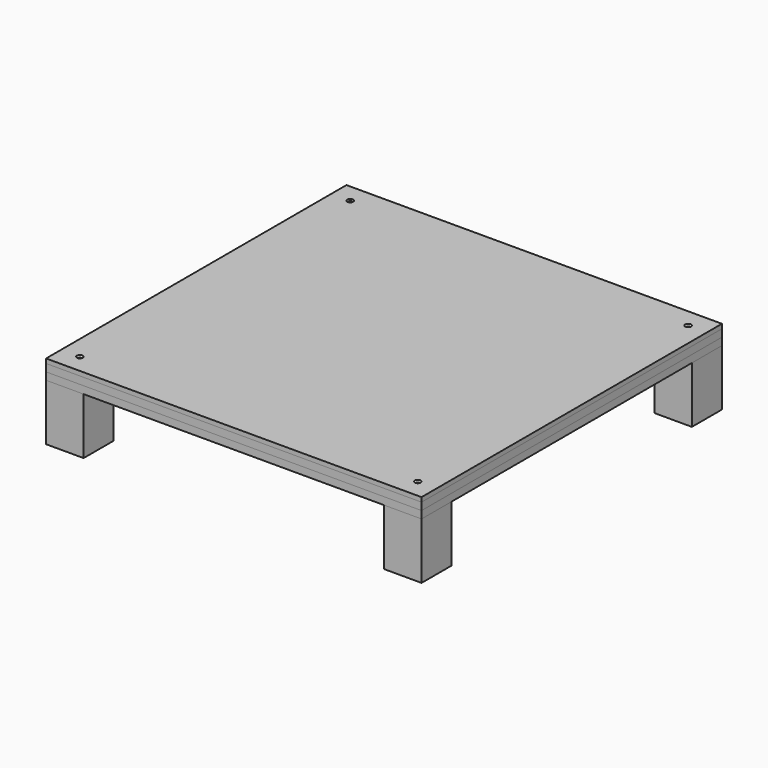
from build123d import *

# Parameters (mm, degrees)
F1_W            = 254
F1_H            = 254
F2_DEPTH        = 4.99999
F0_W            = 254
F0_H            = 254
F3_DEPTH        = 2.999994
F4_DEPTH        = 4.99999
F5_W            = 25.4
F5_H            = 25.4
F6_DEPTH        = 38.1
F7_W            = 25.4
F7_H            = 25.4
F8_DEPTH        = 38.1
F9_W            = 25.4
F9_H            = 25.4
F10_DEPTH       = 38.1
F11_W           = 25.4
F11_H           = 25.4
F12_DEPTH       = 38.1
F14_D           = 2.4892
F14_DEPTH       = 25.4
F14_TIP         = 0.7478311264
F14_2_D         = 2.4892
F14_2_DEPTH     = 25.4
F14_2_TIP       = 0.7478311264
F14_3_D         = 2.4892
F14_3_DEPTH     = 25.4
F14_3_TIP       = 0.7478311264
F14_4_D         = 2.4892
F14_4_DEPTH     = 25.4
F14_4_TIP       = 0.7478311264
F16_D           = 2.4892
F16_DEPTH       = 3.999992
F16_CSINK_D     = 3.999992
F16_CSINK_ANGLE = 90
F16_TIP         = 0.7478311264
F18_D           = 2.00000108
F18_DEPTH       = 25.4
F18_TIP         = 0.6008609435
F18_2_D         = 2.00000108
F18_2_DEPTH     = 25.4
F18_2_TIP       = 0.6008609435
F18_3_D         = 2.00000108
F18_3_DEPTH     = 25.4
F18_3_TIP       = 0.6008609435
F18_4_D         = 2.00000108
F18_4_DEPTH     = 25.4
F18_4_TIP       = 0.6008609435
F20_D           = 2.00000108
F20_DEPTH       = 3.999992
F20_CSINK_D     = 3.999992
F20_CSINK_ANGLE = 90
F20_TIP         = 0.6008609435
F22_D           = 2
F22_DEPTH       = 25.4
F22_TIP         = 0.600860619
F22_2_D         = 2
F22_2_DEPTH     = 25.4
F22_2_TIP       = 0.600860619
F22_3_D         = 2
F22_3_DEPTH     = 25.4
F22_3_TIP       = 0.600860619
F22_4_D         = 2
F22_4_DEPTH     = 25.4
F22_4_TIP       = 0.600860619
F23_D           = 2
F23_DEPTH       = 25.4
F23_TIP         = 0.600860619
F23_2_D         = 2
F23_2_DEPTH     = 25.4
F23_2_TIP       = 0.600860619
F23_3_D         = 2
F23_3_DEPTH     = 25.4
F23_3_TIP       = 0.600860619
F23_4_D         = 2
F23_4_DEPTH     = 25.4
F23_4_TIP       = 0.600860619
F24_D           = 2
F24_DEPTH       = 4
F24_CSINK_D     = 4
F24_CSINK_ANGLE = 90
F24_TIP         = 0.600860619
F25_D           = 2
F25_DEPTH       = 4
F25_CSINK_D     = 4
F25_CSINK_ANGLE = 90
F25_TIP         = 0.600860619
F26_W           = 203.2
F26_H           = 203.2
F27_DEPTH       = 5
F28_W           = 25.4
F28_H           = 25.4
F29_DEPTH       = 5
F30_W           = 25.4
F30_H           = 25.4
F31_DEPTH       = 5
F32_W           = 25.4
F32_H           = 25.4
F33_DEPTH       = 5
F34_W           = 25.4
F34_H           = 25.4
F35_DEPTH       = 5
F36_W           = 25.4
F36_H           = 25.4
F37_DEPTH       = 5


with BuildPart() as f2:
    # F1 (on Top) → F2 (new body)
    with BuildSketch(Plane.XY):
        Rectangle(F1_W, F1_H)
    extrude(amount=-F2_DEPTH)


with BuildPart() as f3:
    # F0 (on Top) → F3 (new body)
    with BuildSketch(Plane.XY):
        Rectangle(F0_W, F0_H)
    extrude(amount=F3_DEPTH)

    # F14#2
    with Locations(Plane.XY.offset(2.999994)):
        with Locations((-114.3, 114.3)):
            Hole(F14_2_D / 2, depth=F14_2_DEPTH)
            with Locations((0, 0, -(F14_2_DEPTH + F14_2_TIP / 2))):  # 118° drill point
                Cone(0, F14_2_D / 2, F14_2_TIP, mode=Mode.SUBTRACT)

    # F16
    with Locations(Plane.XY.offset(2.999994)):
        with Locations((-114.3, 114.3)):
            CounterSinkHole(F16_D / 2, F16_CSINK_D / 2, depth=F16_DEPTH, counter_sink_angle=F16_CSINK_ANGLE)
            with Locations((0, 0, -(F16_DEPTH + F16_TIP / 2))):  # 118° drill point
                Cone(0, F16_D / 2, F16_TIP, mode=Mode.SUBTRACT)

    # F18#2
    with Locations(Plane.XY.offset(2.999994)):
        with Locations((114.3, 114.3)):
            Hole(F18_2_D / 2, depth=F18_2_DEPTH)
            with Locations((0, 0, -(F18_2_DEPTH + F18_2_TIP / 2))):  # 118° drill point
                Cone(0, F18_2_D / 2, F18_2_TIP, mode=Mode.SUBTRACT)

    # F20
    with Locations(Plane.XY.offset(2.999994)):
        with Locations((114.3, 114.3)):
            CounterSinkHole(F20_D / 2, F20_CSINK_D / 2, depth=F20_DEPTH, counter_sink_angle=F20_CSINK_ANGLE)
            with Locations((0, 0, -(F20_DEPTH + F20_TIP / 2))):  # 118° drill point
                Cone(0, F20_D / 2, F20_TIP, mode=Mode.SUBTRACT)

    # F22#2
    with Locations(Plane.XY.offset(2.999994)):
        with Locations((-114.3, -114.3)):
            Hole(F22_2_D / 2, depth=F22_2_DEPTH)
            with Locations((0, 0, -(F22_2_DEPTH + F22_2_TIP / 2))):  # 118° drill point
                Cone(0, F22_2_D / 2, F22_2_TIP, mode=Mode.SUBTRACT)

    # F23#2
    with Locations(Plane.XY.offset(2.999994)):
        with Locations((114.3, -114.3)):
            Hole(F23_2_D / 2, depth=F23_2_DEPTH)
            with Locations((0, 0, -(F23_2_DEPTH + F23_2_TIP / 2))):  # 118° drill point
                Cone(0, F23_2_D / 2, F23_2_TIP, mode=Mode.SUBTRACT)

    # F24
    with Locations(Plane.XY.offset(2.999994)):
        with Locations((114.3, -114.3)):
            CounterSinkHole(F24_D / 2, F24_CSINK_D / 2, depth=F24_DEPTH, counter_sink_angle=F24_CSINK_ANGLE)
            with Locations((0, 0, -(F24_DEPTH + F24_TIP / 2))):  # 118° drill point
                Cone(0, F24_D / 2, F24_TIP, mode=Mode.SUBTRACT)

    # F25
    with Locations(Plane.XY.offset(2.999994)):
        with Locations((-114.3, -114.3)):
            CounterSinkHole(F25_D / 2, F25_CSINK_D / 2, depth=F25_DEPTH, counter_sink_angle=F25_CSINK_ANGLE)
            with Locations((0, 0, -(F25_DEPTH + F25_TIP / 2))):  # 118° drill point
                Cone(0, F25_D / 2, F25_TIP, mode=Mode.SUBTRACT)


with BuildPart() as f4:
    # F4 (new): a face of the model
    f4_faces = [f2.part.faces().sort_by_distance(p)[0] for p in [
        (0, 0, -4.99999),
    ]]
    extrude(f4_faces, amount=F4_DEPTH)

    # F14#3
    with Locations(Plane.XY.offset(2.999994)):
        with Locations((-114.3, 114.3)):
            Hole(F14_3_D / 2, depth=F14_3_DEPTH)
            with Locations((0, 0, -(F14_3_DEPTH + F14_3_TIP / 2))):  # 118° drill point
                Cone(0, F14_3_D / 2, F14_3_TIP, mode=Mode.SUBTRACT)

    # F18#3
    with Locations(Plane.XY.offset(2.999994)):
        with Locations((114.3, 114.3)):
            Hole(F18_3_D / 2, depth=F18_3_DEPTH)
            with Locations((0, 0, -(F18_3_DEPTH + F18_3_TIP / 2))):  # 118° drill point
                Cone(0, F18_3_D / 2, F18_3_TIP, mode=Mode.SUBTRACT)

    # F22#3
    with Locations(Plane.XY.offset(2.999994)):
        with Locations((-114.3, -114.3)):
            Hole(F22_3_D / 2, depth=F22_3_DEPTH)
            with Locations((0, 0, -(F22_3_DEPTH + F22_3_TIP / 2))):  # 118° drill point
                Cone(0, F22_3_D / 2, F22_3_TIP, mode=Mode.SUBTRACT)

    # F23#3
    with Locations(Plane.XY.offset(2.999994)):
        with Locations((114.3, -114.3)):
            Hole(F23_3_D / 2, depth=F23_3_DEPTH)
            with Locations((0, 0, -(F23_3_DEPTH + F23_3_TIP / 2))):  # 118° drill point
                Cone(0, F23_3_D / 2, F23_3_TIP, mode=Mode.SUBTRACT)


with BuildPart() as f6:
    # F5 (on face) → F6 (new body)
    with BuildSketch(Plane(origin=(0, 0, -9.99998), x_dir=(1, 0, 0), z_dir=(0, 0, -1))):
        with Locations((-114.3, 114.3)):
            Rectangle(F5_W, F5_H)
    extrude(amount=F6_DEPTH)

    # F22#4
    with Locations(Plane.XY.offset(2.999994)):
        with Locations((-114.3, -114.3)):
            Hole(F22_4_D / 2, depth=F22_4_DEPTH)
            with Locations((0, 0, -(F22_4_DEPTH + F22_4_TIP / 2))):  # 118° drill point
                Cone(0, F22_4_D / 2, F22_4_TIP, mode=Mode.SUBTRACT)


with BuildPart() as f8:
    # F7 (on face) → F8 (new body)
    with BuildSketch(Plane(origin=(0, 0, -9.99998), x_dir=(1, 0, 0), z_dir=(0, 0, -1))):
        with Locations((114.3, 114.3)):
            Rectangle(F7_W, F7_H)
    extrude(amount=F8_DEPTH)

    # F23#4
    with Locations(Plane.XY.offset(2.999994)):
        with Locations((114.3, -114.3)):
            Hole(F23_4_D / 2, depth=F23_4_DEPTH)
            with Locations((0, 0, -(F23_4_DEPTH + F23_4_TIP / 2))):  # 118° drill point
                Cone(0, F23_4_D / 2, F23_4_TIP, mode=Mode.SUBTRACT)


with BuildPart() as f10:
    # F9 (on face) → F10 (new body)
    with BuildSketch(Plane(origin=(0, 0, -9.99998), x_dir=(1, 0, 0), z_dir=(0, 0, -1))):
        with Locations((114.3, -114.3)):
            Rectangle(F9_W, F9_H)
    extrude(amount=F10_DEPTH)

    # F18#4
    with Locations(Plane.XY.offset(2.999994)):
        with Locations((114.3, 114.3)):
            Hole(F18_4_D / 2, depth=F18_4_DEPTH)
            with Locations((0, 0, -(F18_4_DEPTH + F18_4_TIP / 2))):  # 118° drill point
                Cone(0, F18_4_D / 2, F18_4_TIP, mode=Mode.SUBTRACT)


with BuildPart() as f12:
    # F11 (on face) → F12 (new body)
    with BuildSketch(Plane(origin=(0, 0, -9.99998), x_dir=(1, 0, 0), z_dir=(0, 0, -1))):
        with Locations((-114.3, -114.3)):
            Rectangle(F11_W, F11_H)
    extrude(amount=F12_DEPTH)

    # F14#4
    with Locations(Plane.XY.offset(2.999994)):
        with Locations((-114.3, 114.3)):
            Hole(F14_4_D / 2, depth=F14_4_DEPTH)
            with Locations((0, 0, -(F14_4_DEPTH + F14_4_TIP / 2))):  # 118° drill point
                Cone(0, F14_4_D / 2, F14_4_TIP, mode=Mode.SUBTRACT)


with BuildPart() as f2_1:
    add(f2.part)

    # F14
    with Locations(Plane.XY.offset(2.999994)):
        with Locations((-114.3, 114.3)):
            Hole(F14_D / 2, depth=F14_DEPTH)
            with Locations((0, 0, -(F14_DEPTH + F14_TIP / 2))):  # 118° drill point
                Cone(0, F14_D / 2, F14_TIP, mode=Mode.SUBTRACT)

    # F18
    with Locations(Plane.XY.offset(2.999994)):
        with Locations((114.3, 114.3)):
            Hole(F18_D / 2, depth=F18_DEPTH)
            with Locations((0, 0, -(F18_DEPTH + F18_TIP / 2))):  # 118° drill point
                Cone(0, F18_D / 2, F18_TIP, mode=Mode.SUBTRACT)

    # F22
    with Locations(Plane.XY.offset(2.999994)):
        with Locations((-114.3, -114.3)):
            Hole(F22_D / 2, depth=F22_DEPTH)
            with Locations((0, 0, -(F22_DEPTH + F22_TIP / 2))):  # 118° drill point
                Cone(0, F22_D / 2, F22_TIP, mode=Mode.SUBTRACT)

    # F23
    with Locations(Plane.XY.offset(2.999994)):
        with Locations((114.3, -114.3)):
            Hole(F23_D / 2, depth=F23_DEPTH)
            with Locations((0, 0, -(F23_DEPTH + F23_TIP / 2))):  # 118° drill point
                Cone(0, F23_D / 2, F23_TIP, mode=Mode.SUBTRACT)


with BuildPart() as f27_tool:
    # F26 (on face) → F27 (new body)
    with BuildSketch(Plane.XY):
        Rectangle(F26_W, F26_H)
    extrude(amount=-F27_DEPTH)


with BuildPart() as f2_2:
    add(f2_1.part)

    # F27: cut by f27_tool
    add(f27_tool.part, mode=Mode.SUBTRACT)


with BuildPart() as f4_1:
    add(f4.part)

    # F27: cut by f27_tool
    add(f27_tool.part, mode=Mode.SUBTRACT)


with BuildPart() as f29:
    # F28 (on face) → F29 (new body)
    with BuildSketch(Plane.XY):
        with Locations((-12.7, -12.7)):
            Rectangle(F28_W, F28_H)
    extrude(amount=-F29_DEPTH)


with BuildPart() as f31:
    # F30 (on face) → F31 (new body)
    with BuildSketch(Plane.XY):
        with Locations((-12.7, 12.7)):
            Rectangle(F30_W, F30_H)
    extrude(amount=-F31_DEPTH)


with BuildPart() as f33:
    # F32 (on face) → F33 (new body)
    with BuildSketch(Plane.XY):
        with Locations((12.7, -12.7)):
            Rectangle(F32_W, F32_H)
    extrude(amount=-F33_DEPTH)


with BuildPart() as f35:
    # F34 (on face) → F35 (new body)
    with BuildSketch(Plane.XY):
        with Locations((38.1, -38.1)):
            Rectangle(F34_W, F34_H)
    extrude(amount=-F35_DEPTH)


with BuildPart() as f37:
    # F36 (on face) → F37 (new body)
    with BuildSketch(Plane.XY):
        with Locations((12.7, 12.7)):
            Rectangle(F36_W, F36_H)
    extrude(amount=-F37_DEPTH)


with BuildPart() as f38_1:
    # F38: copy of F37
    add(f37.part.moved(Location((25.4, 25.4, 0))))


with BuildPart() as f39_1:
    # F39: copy of F38_1
    add(f38_1.part.moved(Location((25.4, 25.4, 0))))


with BuildPart() as f40_1:
    # F40: copy of F39_1
    add(f39_1.part.moved(Location((25.4, 25.4, 0))))


with BuildPart() as f41_1:
    # F41: copy of F29
    add(f29.part.moved(Location((-25.4, -25.4, 0))))


with BuildPart() as f42_1:
    # F42: copy of F41_1
    add(f41_1.part.moved(Location((-25.4, -25.4, 0))))


with BuildPart() as f43_1:
    # F43: copy of F42_1
    add(f42_1.part.moved(Location((-25.4, -25.4, 0))))


with BuildPart() as f44_1:
    # F44: copy of F31
    add(f31.part.moved(Location((-25.4, 25.4, 0))))


with BuildPart() as f45_1:
    # F45: copy of F44_1
    add(f44_1.part.moved(Location((-25.4, 25.4, 0))))


with BuildPart() as f46_1:
    # F46: copy of F45_1
    add(f45_1.part.moved(Location((-25.4, 25.4, 0))))


with BuildPart() as f47_1:
    # F47: copy of F35
    add(f35.part.moved(Location((25.4, -25.4, 0))))


with BuildPart() as f48_1:
    # F48: copy of F47_1
    add(f47_1.part.moved(Location((25.4, -25.4, 0))))


with BuildPart() as f49_1:
    # F49: copy of F48_1
    add(f48_1.part.moved(Location((-50.8, 0, 0))))


with BuildPart() as f50_1:
    # F50: copy of F49_1
    add(f49_1.part.moved(Location((-50.8, 0, 0))))


with BuildPart() as f51_1:
    # F51: copy of F50_1
    add(f50_1.part.moved(Location((-50.8, 0, 0))))


with BuildPart() as f52_1:
    # F52: copy of F51_1
    add(f51_1.part.moved(Location((0, 50.8, 0))))


with BuildPart() as f53_1:
    # F53: copy of F51_1
    add(f51_1.part.moved(Location((0, 50.8, 0))))


with BuildPart() as f55_1:
    # F55: copy of F53_1
    add(f53_1.part.moved(Location((0, 50.8, 0))))


with BuildPart() as f56_1:
    # F56: copy of F50_1
    add(f50_1.part.moved(Location((0, 50.8, 0))))


with BuildPart() as f56_2:
    # F56: copy of F4
    add(f4_1.part.moved(Location((0, 50.8, 0))))


with BuildPart() as f58_1:
    # F58: copy of F46_1
    add(f46_1.part.moved(Location((0, -50.8, 0))))


with BuildPart() as f59_1:
    # F59: copy of F58_1
    add(f58_1.part.moved(Location((0, -50.8, 0))))


with BuildPart() as f60_1:
    # F60: copy of F59_1
    add(f59_1.part.moved(Location((0, -50.8, 0))))


with BuildPart() as f61_1:
    # F61: copy of F58_1
    add(f58_1.part.moved(Location((101.6, 0, 0))))


with BuildPart() as f61_2:
    # F61: copy of F44_1
    add(f44_1.part.moved(Location((101.6, 0, 0))))


with BuildPart() as f62_1:
    # F62: copy of F61_1
    add(f61_1.part.moved(Location((0, 50.8, 0))))


with BuildPart() as f63_1:
    # F63: copy of F62_1
    add(f62_1.part.moved(Location((-50.8, 0, 0))))


with BuildPart() as f64_1:
    # F64: copy of F62_1
    add(f62_1.part.moved(Location((50.8, 0, 0))))


with BuildPart() as f65_1:
    # F65: copy of F63_1
    add(f63_1.part.moved(Location((25.4, -25.4, 0))))


with BuildPart() as f66_1:
    # F66: copy of F65_1
    add(f65_1.part.moved(Location((50.8, 0, 0))))


with BuildPart() as f67_1:
    # F67: copy of F66_1
    add(f66_1.part.moved(Location((50.8, 0, 0))))


with BuildPart() as f68_1:
    # F68: copy of F67_1
    add(f67_1.part.moved(Location((0, -50.8, 0))))


with BuildPart() as f69_1:
    # F69: copy of F68_1
    add(f68_1.part.moved(Location((0, -50.8, 0))))


with BuildPart() as f70_1:
    # F70: copy of F69_1
    add(f69_1.part.moved(Location((-25.4, 25.4, 0))))


with BuildPart() as f71_1:
    # F71: copy of F70_1
    add(f70_1.part.moved(Location((-25.4, 25.4, 0))))


with BuildPart() as f72_1:
    # F72: copy of F69_1
    add(f69_1.part.moved(Location((-76.2, -25.4, 0))))


with BuildPart() as f73_1:
    # F73: copy of F72_1
    add(f72_1.part.moved(Location((-50.8, 0, 0))))


with BuildPart() as f74_1:
    # F74: copy of F40_1
    add(f40_1.part.moved(Location((0, -50.8, 0))))


with BuildPart() as f75_1:
    # F75: copy of F74_1
    add(f74_1.part.moved(Location((0, -50.8, 0))))


with BuildPart() as f76_1:
    # F76: copy of F75_1
    add(f75_1.part.moved(Location((0, -50.8, 0))))


with BuildPart() as f77_1:
    # F77: copy of F76_1
    add(f76_1.part.moved(Location((-25.4, -25.4, 0))))


with BuildPart() as f78_1:
    # F78: copy of F77_1
    add(f77_1.part.moved(Location((0, 50.8, 0))))


with BuildPart() as f79_1:
    # F79: copy of F78_1
    add(f78_1.part.moved(Location((0, 50.8, 0))))


with BuildPart() as f80_1:
    # F80: copy of F77_1
    add(f77_1.part.moved(Location((-25.4, 25.4, 0))))


with BuildPart() as f81_1:
    # F81: copy of F80_1
    add(f80_1.part.moved(Location((0, 50.8, 0))))


with BuildPart() as f82_1:
    # F82: copy of F81_1
    add(f81_1.part.moved(Location((0, 101.6, 0))))


with BuildPart() as f83_1:
    # F83: copy of F82_1
    add(f82_1.part.moved(Location((-25.4, -25.4, 0))))


with BuildPart() as f84_1:
    # F84: copy of F83_1
    add(f83_1.part.moved(Location((0, -101.6, 0))))


with BuildPart() as f85_1:
    # F85: copy of F84_1
    add(f84_1.part.moved(Location((0, -50.8, 0))))


with BuildPart() as f86_1:
    # F86: copy of F85_1
    add(f85_1.part.moved(Location((-25.4, 25.4, 0))))


with BuildPart() as f87_1:
    # F87: copy of F86_1
    add(f86_1.part.moved(Location((0, 101.6, 0))))


with BuildPart() as f88_1:
    # F88: copy of F87_1
    add(f87_1.part.moved(Location((0, 50.8, 0))))


with BuildPart() as f89_1:
    # F89: copy of F88_1
    add(f88_1.part.moved(Location((-25.4, -25.4, 0))))


with BuildPart() as f90_1:
    # F90: copy of F89_1
    add(f89_1.part.moved(Location((0, -50.8, 0))))


with BuildPart() as f91_1:
    # F91: copy of F90_1
    add(f90_1.part.moved(Location((0, -101.6, 0))))


with BuildPart() as f92_1:
    # F92: copy of F91_1
    add(f91_1.part.moved(Location((-50.8, 50.8, 0))))


with BuildPart() as f93_1:
    # F93: copy of F92_1
    add(f92_1.part.moved(Location((0, 50.8, 0))))


with BuildPart() as f94_1:
    # F94: copy of F93_1
    add(f93_1.part.moved(Location((0, 50.8, 0))))


with BuildPart() as f95_1:
    # F95: copy of F94_1
    add(f94_1.part.moved(Location((25.4, 25.4, 0))))


with BuildPart() as f96_1:
    # F96: copy of F95_1
    add(f95_1.part.moved(Location((0, -50.8, 0))))


with BuildPart() as f97_1:
    # F97: copy of F96_1
    add(f96_1.part.moved(Location((0, -50.8, 0))))


with BuildPart() as f98_1:
    # F98: copy of F70_1
    add(f70_1.part.moved(Location((-101.6, 0, 0))))


solid = Compound([f3.part, f6.part, f8.part, f10.part, f12.part, f2_2.part, f4_1.part, f29.part, f31.part, f33.part, f35.part, f37.part, f38_1.part, f39_1.part, f40_1.part, f41_1.part, f42_1.part, f43_1.part, f44_1.part, f45_1.part, f46_1.part, f47_1.part, f48_1.part, f49_1.part, f50_1.part, f51_1.part, f53_1.part, f55_1.part, f56_1.part, f58_1.part, f59_1.part, f60_1.part, f61_1.part, f61_2.part, f62_1.part, f63_1.part, f64_1.part, f65_1.part, f66_1.part, f67_1.part, f68_1.part, f69_1.part, f70_1.part, f71_1.part, f72_1.part, f73_1.part, f74_1.part, f75_1.part, f76_1.part, f77_1.part, f78_1.part, f79_1.part, f80_1.part, f81_1.part, f82_1.part, f83_1.part, f84_1.part, f85_1.part, f86_1.part, f87_1.part, f88_1.part, f89_1.part, f90_1.part, f91_1.part, f92_1.part, f93_1.part, f94_1.part, f95_1.part, f96_1.part, f97_1.part, f98_1.part])
